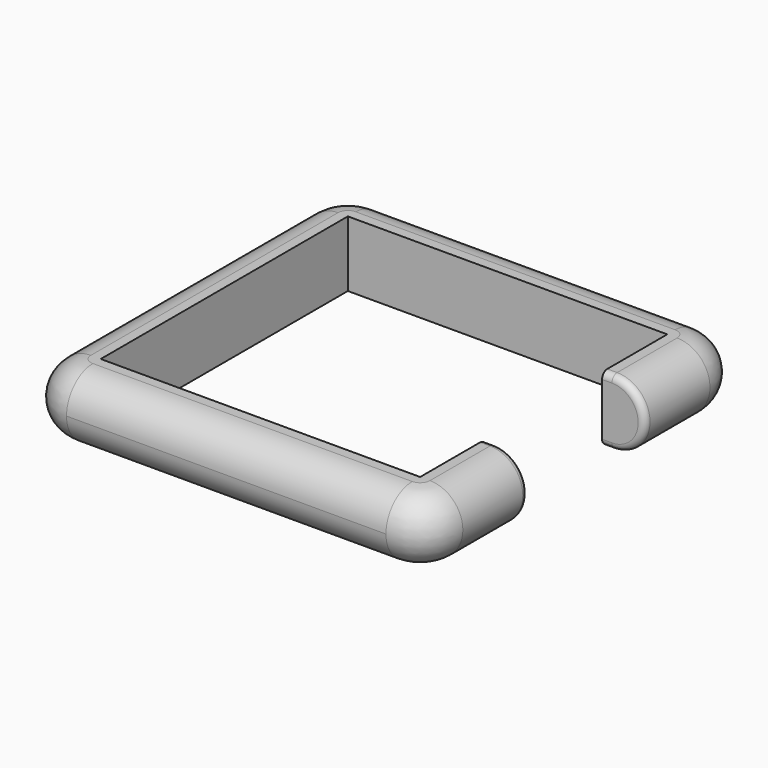
from build123d import *

# Parameters (mm, degrees)
F1_DEPTH  = 617.22
F0_W      = 19.05
F0_H      = 127
F2_DEPTH  = 596.9
F3_DEPTH  = 152.4
F6_ANGLE  = 90
F12_ANGLE = -90
F18_ANGLE = 90
F19_ANGLE = 90
F23_ANGLE = 90
F24_ANGLE = 90
F25_DEPTH = 5.08
F26_DEPTH = 5.08
F27_R     = 12.7


with BuildPart() as f1:
    # F0 (on Front) → F1 (new body)
    with BuildSketch(Plane.XZ):
        with BuildLine():
            Line((19.05, 127), (19.05, 63.5))
            Line((19.05, 63.5), (82.55, 63.5))
            ThreePointArc((82.55, 63.5), (63.9512806053, 108.4012806053), (19.05, 127))
        make_face()
        with BuildLine():
            Line((19.05, 63.5), (19.05, 0))
            ThreePointArc((19.05, 0), (63.9512806053, 18.5987193947), (82.55, 63.5))
            Line((82.55, 63.5), (19.05, 63.5))
        make_face()
        Polygon((0, 127), (0, 0), (19.05, 0), (19.05, 63.5), (19.05, 127), align=None)
    extrude(amount=F1_DEPTH)


with BuildPart() as f2:
    # F0 (on Front) → F2 (new body)
    with BuildSketch(Plane.XZ):
        with Locations((249.8001466751, 63.5)):
            Rectangle(F0_W, F0_H)
        with BuildLine():
            ThreePointArc((240.2751466751, 127), (195.3738660698, 108.4012806053), (176.7751466751, 63.5))
            ThreePointArc((176.7751466751, 63.5), (195.3738660698, 18.5987193947), (240.2751466751, 0))
            Line((240.2751466751, 0), (240.2751466751, 127))
        make_face()
    extrude(amount=F2_DEPTH)


with BuildPart() as f3:
    # F0 (on Front) → F3 (new body)
    with BuildSketch(Plane.XZ):
        with BuildLine():
            ThreePointArc((-240.2751466751, 0), (-195.3738660698, 18.5987193947), (-176.7751466751, 63.5))
            ThreePointArc((-176.7751466751, 63.5), (-195.3738660698, 108.4012806053), (-240.2751466751, 127))
            Line((-240.2751466751, 127), (-240.2751466751, 0))
        make_face()
        with Locations((-249.8001466751, 63.5)):
            Rectangle(F0_W, F0_H)
    extrude(amount=F3_DEPTH)


with BuildPart() as f4_1:
    # F4: copy of F3
    add(f3.part.moved(Location((127, 0, 0))))


with BuildPart() as f5_1:
    # F5: copy of F1
    add(f1.part.moved(Location((127, 127, 254))))


with BuildPart() as f5_1_1:
    # F6: moved
    add(f5_1.part.rotate(Axis((127, 127, 317.5), (0, 0, 1)), F6_ANGLE))


with BuildPart() as f5_1_2:
    # F9: moved
    add(f5_1_1.part.moved(Location((0, -127, -254))))


with BuildPart() as f5_1_3:
    # F11: moved
    add(f5_1_2.part.moved(Location((132.3251466751, 0, 0))))


with BuildPart() as f1_1:
    # F12: moved
    add(f1.part.rotate(Axis((0, -617.22, 63.5), (0, 0, 1)), F12_ANGLE))


with BuildPart() as f1_2:
    # F14: moved
    add(f1_1.part.moved(Location((0, 20.32, 0))))


with BuildPart() as f1_3:
    # F16: moved
    add(f1_2.part.moved(Location((259.3251466751, 0, 0))))


    add(f2.part)  # F18 merges F2
    # F2_face1 (on face) → F18 (revolve)
    with BuildSketch(Plane(origin=(223.4065289788, -596.9, 63.5), x_dir=(1, 0, 0), z_dir=(0, -1, 0))):
        with BuildLine():
            Line((35.9186176963, 63.5), (16.8686176963, 63.5))
            ThreePointArc((16.8686176963, 63.5), (-46.6313823037, 0), (16.8686176963, -63.5))
            Line((16.8686176963, -63.5), (35.9186176963, -63.5))
            Line((35.9186176963, -63.5), (35.9186176963, 63.5))
        make_face()
    revolve(axis=Axis((259.3251466751, -596.9, 63.5), (0, 0, 1)), revolution_arc=F18_ANGLE)


    add(f5_1_3.part)  # F19 merges F5_1
    # F0 (on Front) → F19 (revolve)
    with BuildSketch(Plane.XZ):
        with Locations((249.8001466751, 63.5)):
            Rectangle(F0_W, F0_H)
        with BuildLine():
            ThreePointArc((240.2751466751, 127), (195.3738660698, 108.4012806053), (176.7751466751, 63.5))
            ThreePointArc((176.7751466751, 63.5), (195.3738660698, 18.5987193947), (240.2751466751, 0))
            Line((240.2751466751, 0), (240.2751466751, 127))
        make_face()
    revolve(axis=Axis((259.3251466751, 0, 63.5), (0, 0, -1)), revolution_arc=F19_ANGLE)



with BuildPart() as f4_1_1:
    # F21: moved
    add(f4_1.part.moved(Location((1008.8702933502, -444.5, 0))))


with BuildPart() as f3_1:
    # F22: moved
    add(f3.part.moved(Location((1135.8702933502, 0, 0))))


with BuildPart() as f1_4:
    add(f1_3.part)

    add(f3_1.part)  # F23 merges F3
    # F5_face1 (on face) → F23 (revolve)
    with BuildSketch(Plane(origin=(876.5451466751, 35.9186176963, 63.5), x_dir=(0, 1, 0), z_dir=(1, 0, 0))):
        with BuildLine():
            ThreePointArc((-16.8686176963, -63.5), (46.6313823037, 0), (-16.8686176963, 63.5))
            Line((-16.8686176963, 63.5), (-35.9186176963, 63.5))
            Line((-35.9186176963, 63.5), (-35.9186176963, -63.5))
            Line((-35.9186176963, -63.5), (-16.8686176963, -63.5))
        make_face()
    revolve(axis=Axis((876.5451466751, 0, 63.5), (0, 0, -1)), revolution_arc=F23_ANGLE)


    add(f4_1_1.part)  # F24 merges F4_1
    # F1_face2 (on face) → F24 (revolve)
    with BuildSketch(Plane(origin=(876.5451466751, -632.8186176963, 63.5), x_dir=(0, 1, 0), z_dir=(1, 0, 0))):
        with BuildLine():
            ThreePointArc((16.8686176963, 63.5), (-46.6313823037, 0), (16.8686176963, -63.5))
            Line((16.8686176963, -63.5), (35.9186176963, -63.5))
            Line((35.9186176963, -63.5), (35.9186176963, 63.5))
            Line((35.9186176963, 63.5), (16.8686176963, 63.5))
        make_face()
    revolve(axis=Axis((876.5451466751, -596.9, 63.5), (0, 0, 1)), revolution_arc=F24_ANGLE)

    # F25 (add): a face of the model
    f25_faces = [f1_4.faces().sort_by_distance(p)[0] for p in [
        (912.4637643715, -444.5, 63.5),
    ]]
    extrude(f25_faces, amount=F25_DEPTH)

    # F26 (add): a face of the model
    f26_faces = [f1_4.faces().sort_by_distance(p)[0] for p in [
        (912.4637643715, -152.4, 63.5),
    ]]
    extrude(f26_faces, amount=F26_DEPTH)

    # F27
    f27_edges = [f1_4.edges().sort_by_distance(p)[0] for p in [
        (959.095147, -439.42, 63.5),
        (886.070147, -439.42, 127),
        (886.070147, -439.42, 0),
        (959.095147, -157.48, 63.5),
        (886.070147, -157.48, 127),
        (886.070147, -157.48, 0),
    ]]
    fillet(f27_edges, radius=F27_R)


solid = f1_4.part
